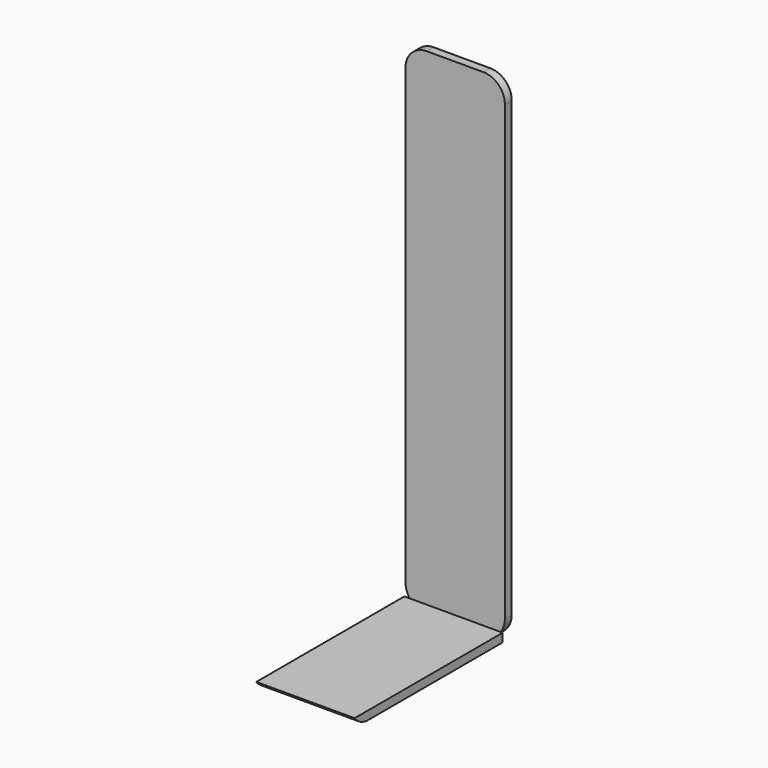
from build123d import *

# Parameters (mm, degrees)
F0_W        = 23.6010048538
F0_H        = 117.7456714213
F1_DEPTH    = 2.032
F2_R        = 5.08
F3_W        = 23.3416529372
F3_H        = 43.9601168036
F4_DEPTH    = 2.032
F5_T1_DEPTH = 43.6616529372


# Not quite as in the source:
# - a fillet or chamfer that OpenCascade refuses, or shapes differently, is made with other operations: its cross-section is extruded or revolved along the edge and cut away or added


with BuildPart() as f1:
    # F0 (on Front) → F1 (new body)
    with BuildSketch(Plane.XZ):
        with Locations((-1.9451379776, -11.8005033582)):
            Rectangle(F0_W, F0_H)
    extrude(amount=-F1_DEPTH)

    # F2
    f2_edges = [f1.edges().sort_by_distance(p)[0] for p in [
        (-13.74564, 1.016, 47.072332),
        (9.855364, 1.016, 47.072332),
        (9.855364, 1.016, -70.673339),
        (-13.74564, 1.016, -70.673339),
    ]]
    fillet(f2_edges, radius=F2_R)

    # F3 (on face) → F4 (join)
    with BuildSketch(Plane(origin=(0, 0, -70.6733390689), x_dir=(1, 0, 0), z_dir=(0, 0, -1))):
        with Locations((-2.3341649212, 21.9800584018)):
            Rectangle(F3_W, F3_H)
    extrude(amount=-F4_DEPTH)

    # F5: fillet of radius 5.08 on 1 edges, made by hand

    # F5_s2 → F5_t1 (cut)
    with BuildSketch(Plane.YZ.offset(-24.1649913898)):
        with BuildLine():
            ThreePointArc((-39.8961168036, -70.6733390689), (-42.1679618688, -70.1370291992), (-43.9601168036, -68.6413390689))
            Line((-43.9601168036, -68.6413390689), (-43.9601168036, -70.6733390689))
            Line((-43.9601168036, -70.6733390689), (-39.8961168036, -70.6733390689))
        make_face()
    extrude(amount=F5_T1_DEPTH, mode=Mode.SUBTRACT)


solid = f1.part
